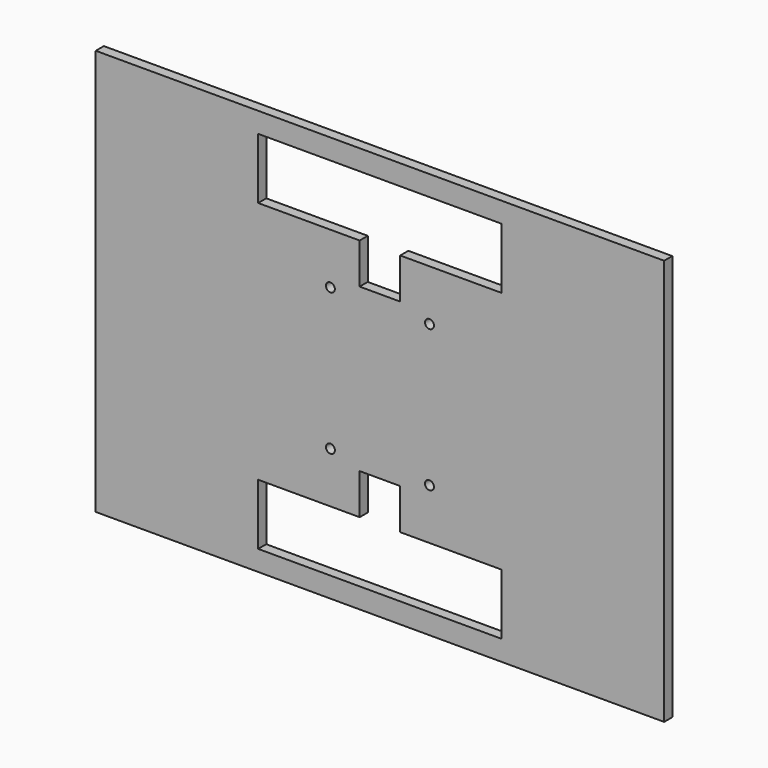
from build123d import *

# Parameters (mm, degrees)
F0_W     = 177.8
F0_H     = 127
F0_R     = 1.397
F1_DEPTH = 3.175


# Not quite as in the source:
# - a feature names something its author has since deleted; it is built from what else it names


with BuildPart() as f1:
    # F0 (on Front) → F1 (new body)
    with BuildSketch(Plane.XZ):
        with Locations((-1.7349944949, 71.7831266678)):
            Rectangle(F0_W, F0_H)
        with Locations((-17.2289944949, 49.5835266678)):
            Circle(F0_R, mode=Mode.SUBTRACT)
        Polygon((-39.8349944949, 14.6331266678), (-39.8349944949, 33.6831266678), (-8.0849944949, 33.6831266678), (-8.0849944949, 46.3831266678), (4.6150055051, 46.3831266678), (4.6150055051, 33.6831266678), (36.3650055051, 33.6831266678), (36.3650055051, 14.6331266678), align=None, mode=Mode.SUBTRACT)
        with Locations((13.7590055051, 49.5835266678)):
            Circle(F0_R, mode=Mode.SUBTRACT)
        with Locations((-17.2289944949, 93.9827266678)):
            Circle(F0_R, mode=Mode.SUBTRACT)
        Polygon((-39.8349944949, 109.8831266678), (-39.8349944949, 128.9331266678), (36.3650055051, 128.9331266678), (36.3650055051, 109.8831266678), (4.6150055051, 109.8831266678), (4.6150055051, 97.1831266678), (-8.0849944949, 97.1831266678), (-8.0849944949, 109.8831266678), align=None, mode=Mode.SUBTRACT)
        with Locations((13.7590055051, 93.9827266678)):
            Circle(F0_R, mode=Mode.SUBTRACT)
    extrude(amount=F1_DEPTH)


solid = f1.part
